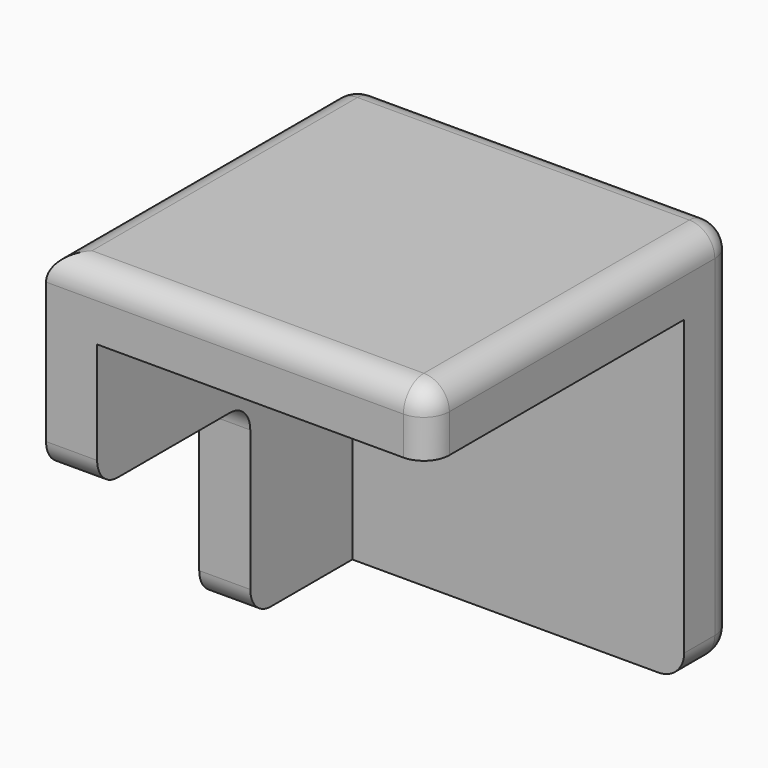
from build123d import *

# Parameters (mm, degrees)
F1_DEPTH     = 30
F3_DEPTH     = 26
F4_R         = 2
F5_T1_DEPTH  = 4
F5_T3_DEPTH  = 14
F5_T5_DEPTH  = 8
F5_T7_DEPTH  = 8
F5_S11_W     = 2
F5_S11_H     = 2
F5_T12_DEPTH = 2
F5_S17_W     = 2
F5_S17_H     = 2
F5_T18_DEPTH = 2


# Not quite as in the source:
# - a fillet or chamfer that OpenCascade refuses, or shapes differently, is made with other operations: its cross-section is extruded or revolved along the edge and cut away or added


with BuildPart() as f1:
    # F0 (on Right) → F1 (new body)
    with BuildSketch(Plane.YZ):
        Polygon((0, -30), (0, 0), (-30, 0), (-30, -15), (-15, -15), (-15, -30), align=None)
    extrude(amount=F1_DEPTH)

    # F2 (on face) → F3 (cut)
    with BuildSketch(Plane.YZ.offset(30)):
        Polygon((-30, -5), (-30, -15), (-15, -15), (-15, -30), (-5, -30), (-5, -5), align=None)
    extrude(amount=-F3_DEPTH, mode=Mode.SUBTRACT)

    # F4
    f4_edges = [f1.edges().sort_by_distance(p)[0] for p in [
        (15, -30, 0),
        (15, 0, 0),
        (0, -15, 0),
        (0, 0, -15),
        (15, 0, -30),
        (30, 0, -15),
        (30, -15, 0),
    ]]
    fillet(f4_edges, radius=F4_R)

    # F5: fillet of radius 2 on 5 edges, made by hand

    # F5_s2 → F5_t1 (join)
    with BuildSketch(Plane.YZ):
        with BuildLine():
            ThreePointArc((-17, -15), (-15.5857864376, -15.5857864376), (-15, -17))
            Line((-15, -17), (-15, -15))
            Line((-15, -15), (-17, -15))
        make_face()
    extrude(amount=F5_T1_DEPTH)

    # F5_s4 → F5_t3 (cut)
    with BuildSketch(Plane.YZ.offset(-5)):
        with BuildLine():
            ThreePointArc((-13, -30), (-14.4142135624, -29.4142135624), (-15, -28))
            Line((-15, -28), (-15, -30))
            Line((-15, -30), (-13, -30))
        make_face()
        with BuildLine():
            ThreePointArc((-30, -13), (-29.4142135624, -14.4142135624), (-28, -15))
            Line((-28, -15), (-30, -15))
            Line((-30, -15), (-30, -13))
        make_face()
    extrude(amount=F5_T3_DEPTH, mode=Mode.SUBTRACT)

    # F5_s6 → F5_t5 (cut)
    with BuildSketch(Plane.XZ.offset(2)):
        with BuildLine():
            ThreePointArc((30, -28), (29.4142135624, -29.4142135624), (28, -30))
            Line((28, -30), (30, -30))
            Line((30, -30), (30, -28))
        make_face()
    extrude(amount=F5_T5_DEPTH, mode=Mode.SUBTRACT)

    # F5_s8 → F5_t7 (cut)
    with BuildSketch(Plane.XY.offset(-10)):
        with BuildLine():
            ThreePointArc((30, -28), (29.4142135624, -29.4142135624), (28, -30))
            Line((28, -30), (30, -30))
            Line((30, -30), (30, -28))
        make_face()
    extrude(amount=F5_T7_DEPTH, mode=Mode.SUBTRACT)


with BuildPart() as f5_tool10:
    # F5_s11 → F5_t12 (new body)
    with BuildSketch(Plane.YZ.offset(28)):
        with Locations((-29, -1)):
            Rectangle(F5_S11_W, F5_S11_H)
    extrude(amount=F5_T12_DEPTH)

    # F5_s13 → F5_t14 (revolve, cut)
    with BuildSketch(Plane(origin=(28, -28, -2), x_dir=(0, 0.7071067812, -0.7071067812), z_dir=(0, -0.7071067812, -0.7071067812))):
        with BuildLine():
            ThreePointArc((0, -2), (2, 0), (0, 2))
            Line((0, 2), (0, -2))
        make_face()
    revolve(axis=Axis((28, -28, -2), (1, 0, 0)), mode=Mode.SUBTRACT)


with BuildPart() as f1_1:
    add(f1.part)

    # F5_t9: cut F5_tool10
    add(f5_tool10.part, mode=Mode.SUBTRACT)


with BuildPart() as f5_tool16:
    # F5_s17 → F5_t18 (new body)
    with BuildSketch(Plane.YZ.offset(28)):
        with Locations((-1, -29)):
            Rectangle(F5_S17_W, F5_S17_H)
    extrude(amount=F5_T18_DEPTH)

    # F5_s19 → F5_t20 (revolve, cut)
    with BuildSketch(Plane(origin=(28, -2, -28), x_dir=(0, -0.7071067812, 0.7071067812), z_dir=(0, 0.7071067812, 0.7071067812))):
        with BuildLine():
            ThreePointArc((0, -2), (2, 0), (0, 2))
            Line((0, 2), (0, -2))
        make_face()
    revolve(axis=Axis((28, -2, -28), (1, 0, 0)), mode=Mode.SUBTRACT)


with BuildPart() as f1_2:
    add(f1_1.part)

    # F5_t15: cut F5_tool16
    add(f5_tool16.part, mode=Mode.SUBTRACT)


solid = f1_2.part
